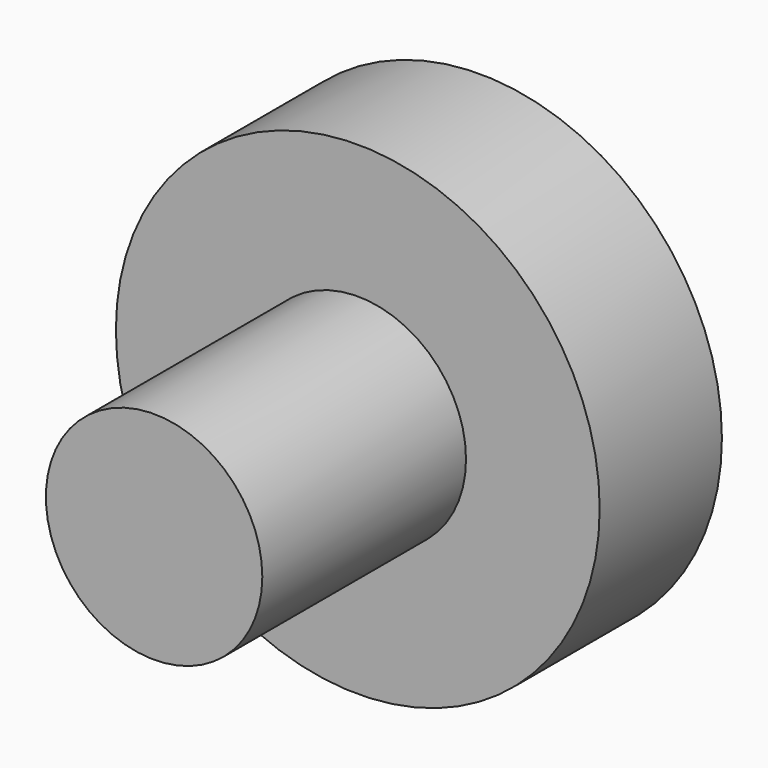
from build123d import *

# Parameters (mm, degrees)
F0_R     = 4.25
F1_DEPTH = 10
F2_R     = 9.5
F2_R_2   = 4.25
F3_DEPTH = 6


# Not quite as in the source:
# - the program builds the solid bodies; features that only make, move or delete a surface that nothing else refers to are left out


with BuildPart() as f1:
    # F0 (on Front) → F1 (new body)
    with BuildSketch(Plane.XZ):
        Circle(F0_R)
    extrude(amount=F1_DEPTH)

    # F2 (on face) → F3 (join)
    with BuildSketch(Plane(origin=(0, 0, 0), x_dir=(-1, 0, 0), z_dir=(0, 1, 0))):
        Circle(F2_R)
        Circle(F2_R_2, mode=Mode.SUBTRACT)
        Circle(F2_R_2)
    extrude(amount=F3_DEPTH)


solid = f1.part
